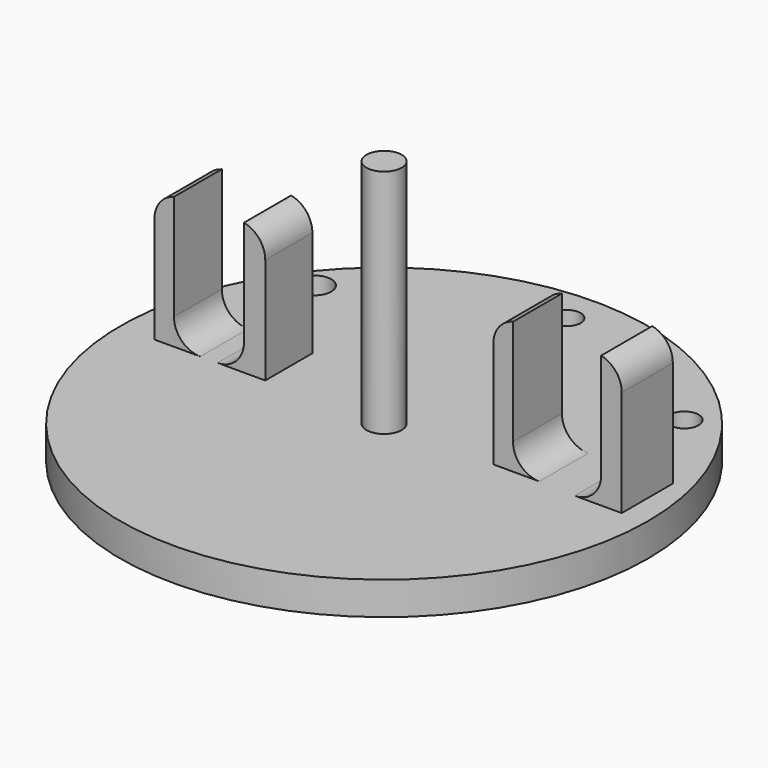
from build123d import *

# Parameters (mm, degrees)
F0_R        = 50.8
F1_DEPTH    = 6.35
F2_R        = 3.3872020891
F3_DEPTH    = 50.8
F4_W        = 3.7956816162
F4_H        = 11.7751168936
F4_W_2      = 3.9597040755
F4_H_2      = 12.2920670431
F4_W_3      = 3.7532411516
F4_H_3      = 11.5020200028
F4_W_4      = 4.1028857231
F4_H_4      = 11.3390376209
F5_DEPTH    = 17.78
F6_R        = 5.08
F7_DEPTH    = 25.4
F8_T1_DEPTH = 36.0204370388
F8_T3_DEPTH = 36.2647510961
F8_T5_DEPTH = 36.3499649547
F8_T7_DEPTH = 37.0667199375
F9_R        = 2.6244366773
F9_R_2      = 2.7684987857
F9_R_3      = 3.2478511369
F10_DEPTH   = 25.4


# Not quite as in the source:
# - a fillet or chamfer that OpenCascade refuses, or shapes differently, is made with other operations: its cross-section is extruded or revolved along the edge and cut away or added


with BuildPart() as f1:
    # F0 (on Top) → F1 (new body)
    with BuildSketch(Plane.XY):
        Circle(F0_R)
    extrude(amount=F1_DEPTH)

    # F2 (on Top) → F3 (join)
    with BuildSketch(Plane.XY):
        Circle(F2_R)
    extrude(amount=F3_DEPTH)

    # F4 (on face) → F5 (join)
    with BuildSketch(Plane.XY.offset(6.35)):
        with Locations((22.9978772923, 5.7736401254)):
            Rectangle(F4_W, F4_H)
        with Locations((44.0967701382, 5.7131922383)):
            Rectangle(F4_W_2, F4_H_2)
        with Locations((-42.1600081027, 5.5507384532)):
            Rectangle(F4_W_3, F4_H_3)
        with Locations((-24.7639858169, 5.4692472622)):
            Rectangle(F4_W_4, F4_H_4)
    extrude(amount=F5_DEPTH)

    # F6
    f6_edges = [f1.edges().sort_by_distance(p)[0] for p in [
        (24.895718, 5.77364, 6.35),
        (42.116918, 5.713192, 6.35),
        (-40.283388, 5.550738, 6.35),
        (-26.815429, 5.469247, 6.35),
    ]]
    fillet(f6_edges, radius=F6_R)

    # F4 (on face) → F7 (join)
    with BuildSketch(Plane.XY.offset(6.35)):
        with Locations((22.9978772923, 5.7736401254)):
            Rectangle(F4_W, F4_H)
        with Locations((44.0967701382, 5.7131922383)):
            Rectangle(F4_W_2, F4_H_2)
        with Locations((-42.1600081027, 5.5507384532)):
            Rectangle(F4_W_3, F4_H_3)
        with Locations((-24.7639858169, 5.4692472622)):
            Rectangle(F4_W_4, F4_H_4)
    extrude(amount=F7_DEPTH)

    # F8: fillet of radius 5.08 on 4 edges, made by hand

    # F8_s2 → F8_t1 (cut)
    with BuildSketch(Plane.XZ.offset(-23.5609569726)):
        with BuildLine():
            ThreePointArc((-40.2833875269, 31.75), (-42.9906301007, 29.9339099153), (-44.0366286784, 26.8463165928))
            Line((-44.0366286784, 26.8463165928), (-44.0366286784, 31.75))
            Line((-44.0366286784, 31.75), (-40.2833875269, 31.75))
        make_face()
    extrude(amount=F8_T1_DEPTH, mode=Mode.SUBTRACT)

    # F8_s4 → F8_t3 (cut)
    with BuildSketch(Plane.XZ.offset(-23.6016228103)):
        with BuildLine():
            ThreePointArc((-26.8154286784, 31.75), (-23.8701622671, 29.9930657457), (-22.7125429553, 26.764857305))
            Line((-22.7125429553, 26.764857305), (-22.7125429553, 31.75))
            Line((-22.7125429553, 31.75), (-26.8154286784, 31.75))
        make_face()
    extrude(amount=F8_T3_DEPTH, mode=Mode.SUBTRACT)

    # F8_s6 → F8_t5 (cut)
    with BuildSketch(Plane.XZ.offset(-23.9486226027)):
        with BuildLine():
            ThreePointArc((24.8957181004, 31.75), (22.1594185349, 29.9400314031), (21.1000364843, 26.8350303878))
            Line((21.1000364843, 26.8350303878), (21.1000364843, 31.75))
            Line((21.1000364843, 31.75), (24.8957181004, 31.75))
        make_face()
    extrude(amount=F8_T5_DEPTH, mode=Mode.SUBTRACT)

    # F8_s8 → F8_t7 (cut)
    with BuildSketch(Plane.XZ.offset(-24.2465522071)):
        with BuildLine():
            ThreePointArc((42.1169181004, 31.75), (44.9650918619, 29.9664489871), (46.0766221759, 26.7950694211))
            Line((46.0766221759, 26.7950694211), (46.0766221759, 31.75))
            Line((46.0766221759, 31.75), (42.1169181004, 31.75))
        make_face()
    extrude(amount=F8_T7_DEPTH, mode=Mode.SUBTRACT)

    # F9 (on face) → F10 (cut)
    with BuildSketch(Plane.XY.offset(6.35)):
        with Locations((0, 43.9927652478)):
            Circle(F9_R)
        with Locations((34.4810411334, 29.0996860713)):
            Circle(F9_R_2)
        with Locations((-36.2776443362, 28.5628065467)):
            Circle(F9_R_3)
    extrude(amount=-F10_DEPTH, mode=Mode.SUBTRACT)


solid = f1.part
